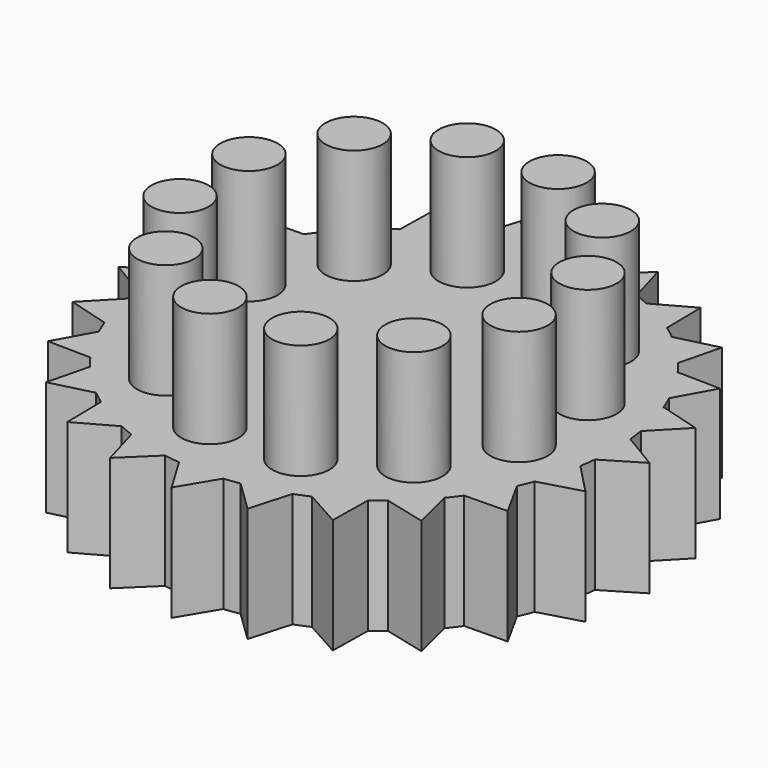
from build123d import *

# Parameters (mm, degrees)
F0_R            = 50.8
F1_DEPTH        = 25.4
F2_R            = 6.35
F3_DEPTH        = 25.4
F3_COPIES_COUNT = 12
F5_DEPTH        = 25.4
F5_COPIES_COUNT = 24


# Not quite as in the source:
# - a pattern or mirror of a feature is missing from the dataset's text; its kind, count and spacing are read off the source's solid


with BuildPart() as f1:
    # F0 (on Top) → F1 (new body)
    with BuildSketch(Plane.XY):
        Circle(F0_R)
    extrude(amount=F1_DEPTH)

    # F2 (on face) → F3 (join)
    with BuildSketch(Plane.XY.offset(25.4)):
        with Locations((-27.5896564126, 26.2101721019)):
            Circle(F2_R)
    f3 = extrude(amount=F3_DEPTH)

    # F3_copies: F3 ×12 about axis
    f3_copies_axis = Axis((0, 0, 0), (0, 0, 1))
    for i in range(1, F3_COPIES_COUNT):
        add(f3.rotate(f3_copies_axis, i * 360 / F3_COPIES_COUNT))

    # F4 (on face) → F5 (join)
    with BuildSketch(Plane.XY.offset(25.4)):
        with BuildLine():
            Line((4.8960702354, 50.5635095326), (0, 58.7265528738))
            Line((0, 58.7265528738), (-4.8960702354, 50.5635095326))
            ThreePointArc((-4.8960702354, 50.5635095326), (0, 50.8), (4.8960702354, 50.5635095326))
        make_face()
        with BuildLine():
            Line((4.8960702354, 50.5635095326), (-4.8960702354, 50.5635095326))
            ThreePointArc((-4.8960702354, 50.5635095326), (-34.1461537515, -37.6122344986), (50.8, 0))
            ThreePointArc((50.8, 0), (37.6122344986, 34.1461537515), (4.8960702354, 50.5635095326))
        make_face()
        with BuildLine():
            ThreePointArc((4.8960702354, 50.5635095326), (0, 50.8), (-4.8960702354, 50.5635095326))
            Line((-4.8960702354, 50.5635095326), (4.8960702354, 50.5635095326))
        make_face()
    f5 = extrude(amount=-F5_DEPTH)

    # F5_copies: F5 ×24 about axis
    f5_copies_axis = Axis((0, 0, 0), (0, 0, 1))
    for i in range(1, F5_COPIES_COUNT):
        add(f5.rotate(f5_copies_axis, i * 360 / F5_COPIES_COUNT))


solid = f1.part
